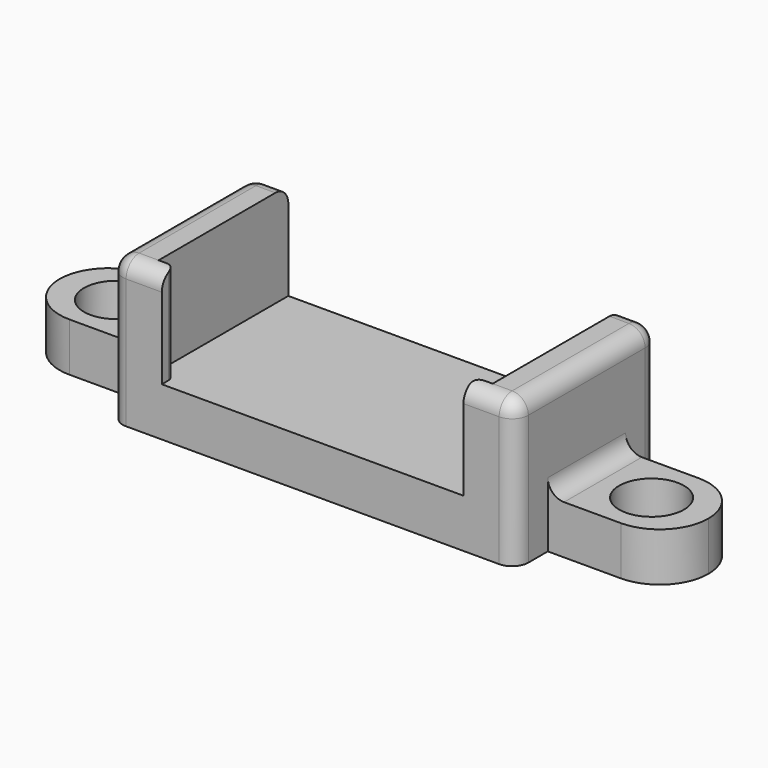
from build123d import *

# Parameters (mm, degrees)
F0_W      = 25
F0_H      = 11
F1_DEPTH  = 9
F2_W      = 20.6
F2_H      = 10
F3_DEPTH  = 6
F4_W      = 18.6
F4_H      = 10
F5_DEPTH  = 6
F8_R      = 0.5
F11_W     = 40
F11_H     = 6
F11_R     = 2
F12_DEPTH = 3
F13_R     = 1
F14_R     = 2.99999


# Not quite as in the source:
# - a fillet or chamfer is up to 0.001 mm smaller than in the source, because OpenCascade refuses the exact size


with BuildPart() as f1:
    # F0 (on Top) → F1 (new body)
    with BuildSketch(Plane.XY):
        Rectangle(F0_W, F0_H)
    extrude(amount=F1_DEPTH)


with BuildPart() as f3:
    # F2 (on Top) → F3 (new body)
    with BuildSketch(Plane.XY):
        Rectangle(F2_W, F2_H)
    extrude(amount=F3_DEPTH)


with BuildPart() as f5:
    # F4 (on Top) → F5 (new body)
    with BuildSketch(Plane.XY):
        Rectangle(F4_W, F4_H)
    extrude(amount=F5_DEPTH)


with BuildPart() as f5_1:
    # F6: moved
    add(f5.part.moved(Location((0, -5, 0))))


with BuildPart() as f3_1:
    add(f3.part)

    # F7: union F5
    add(f5_1.part)

    # F8
    f8_edges = [f3_1.edges().sort_by_distance(p)[0] for p in [
        (-9.3, -5, 3),
        (9.3, -5, 3),
    ]]
    fillet(f8_edges, radius=F8_R)


with BuildPart() as f3_2:
    # F9: moved
    add(f3_1.part.moved(Location((0, 0.5, 3))))


with BuildPart() as f1_1:
    add(f1.part)

    # F10: cut F3
    add(f3_2.part, mode=Mode.SUBTRACT)

    # F11 (on Top) → F12 (join)
    with BuildSketch(Plane.XY):
        Rectangle(F11_W, F11_H)
        with Locations((-16.5, 0)):
            Circle(F11_R, mode=Mode.SUBTRACT)
        with BuildLine():
            ThreePointArc((18.5, 0), (16.5, -2), (14.5, 0))
            ThreePointArc((14.5, 0), (16.5, 2), (18.5, 0))
        make_face(mode=Mode.SUBTRACT)
    extrude(amount=F12_DEPTH)

    # F13
    f13_edges = [f1_1.edges().sort_by_distance(p)[0] for p in [
        (-12.5, 5.5, 4.5),
        (-12.5, -5.5, 4.5),
        (12.5, -5.5, 4.5),
        (12.5, 5.5, 4.5),
        (12.5, 0, 3),
        (-12.5, 0, 3),
        (-12.5, 0, 9),
        (12.5, 0, 9),
        (-11.4, 5.5, 9),
        (11.4, 5.5, 9),
        (10.9, -5.5, 9),
        (-10.9, -5.5, 9),
    ]]
    fillet(f13_edges, radius=F13_R)

    # F14 (radius 3 in the source; OpenCascade refuses exactly that, so slightly less here)
    f14_edges = [f1_1.edges().sort_by_distance(p)[0] for p in [
        (-20, -3, 1.5),
        (-20, 3, 1.5),
        (20, 3, 1.5),
        (20, -3, 1.5),
    ]]
    fillet(f14_edges, radius=F14_R)


solid = f1_1.part
